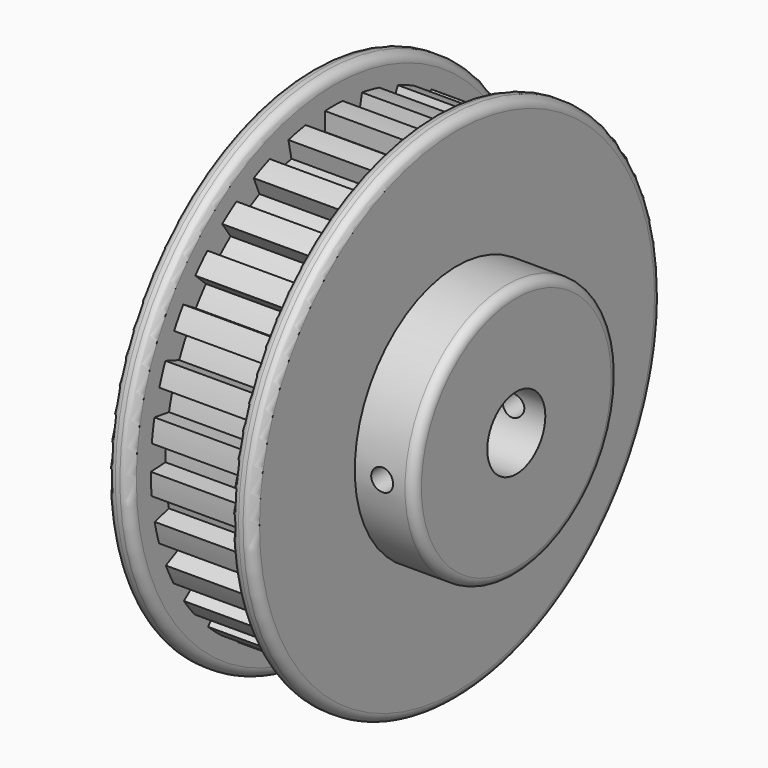
from build123d import *

# Parameters (mm, degrees)
F0_R            = 14
F0_R_2          = 3.975
F1_DEPTH        = 14.5
F2_R            = 23.05
F2_R_2          = 14
F3_DEPTH        = 8
F4_W            = 2.5
F4_H            = 5
F4_W_2          = 11
F8_DEPTH        = 11
F8_COPIES_COUNT = 31
F8_COPIES_ANGLE = 348.39
F9_R            = 1
F10_R           = 1.2
F11_DEPTH       = 25


# Not quite as in the source:
# - a pattern or mirror of a feature is missing from the dataset's text; its kind, count and spacing are read off the source's solid


with BuildPart() as f1:
    # F0 (on Right) → F1 (new body, symmetric)
    with BuildSketch(Plane.YZ):
        Circle(F0_R)
        Circle(F0_R_2, mode=Mode.SUBTRACT)
    extrude(amount=F1_DEPTH, both=True)

    # F2 (on Right) → F3 (join, symmetric)
    with BuildSketch(Plane.YZ):
        Circle(F2_R)
        Circle(F2_R_2, mode=Mode.SUBTRACT)
    extrude(amount=F3_DEPTH, both=True)

    # F4 (on Front) → F5 (revolve)
    with BuildSketch(Plane.XZ):
        with Locations((-6.75, 25.55)):
            Rectangle(F4_W, F4_H)
        with Locations((6.75, 25.55)):
            Rectangle(F4_W, F4_H)
    revolve(axis=Axis((1.1437470717, 0, 0), (1, 0, 0)))

    # F4 (on Front) → F6 (revolve, cut)
    with BuildSketch(Plane.XZ):
        with Locations((0, 25.55)):
            Rectangle(F4_W_2, F4_H)
    revolve(axis=Axis((1.1437470717, 0, 0), (1, 0, 0)), mode=Mode.SUBTRACT)

    # F7 (on face) → F8 (join, through all)
    with BuildSketch(Plane.YZ.offset(-5.5)):
        with BuildLine():
            ThreePointArc((-1.2, 23.0187423636), (0, 23.05), (1.2, 23.0187423636))
            Line((1.2, 23.0187423636), (1.2, 25.0347564847))
            ThreePointArc((1.2, 25.0347564847), (0, 25.0635), (-1.2, 25.0347564847))
            Line((-1.2, 25.0347564847), (-1.2, 23.0187423636))
        make_face()
    f8 = extrude(amount=F8_DEPTH)

    # F8_copies: F8 ×31 about axis
    f8_copies_axis = Axis((0, 0, 0), (-1, 0, 0))
    for i in range(1, F8_COPIES_COUNT):
        add(f8.rotate(f8_copies_axis, i * F8_COPIES_ANGLE / (F8_COPIES_COUNT - 1)))

    # F9
    f9_edges = [f1.edges().sort_by_distance(p)[0] for p in [
        (-5.5, 0, -28.05),
        (5.5, 0, -28.05),
        (-14.5, -14, 0),
        (14.5, -14, 0),
        (-8, 0, -28.05),
        (8, 0, -28.05),
    ]]
    fillet(f9_edges, radius=F9_R)

    # F10 (on Front) → F11 (cut, symmetric)
    with BuildSketch(Plane.XZ):
        with Locations((-11, 0)):
            Circle(F10_R)
        with Locations((11, 0)):
            Circle(F10_R)
    extrude(amount=F11_DEPTH, both=True, mode=Mode.SUBTRACT)


solid = f1.part
